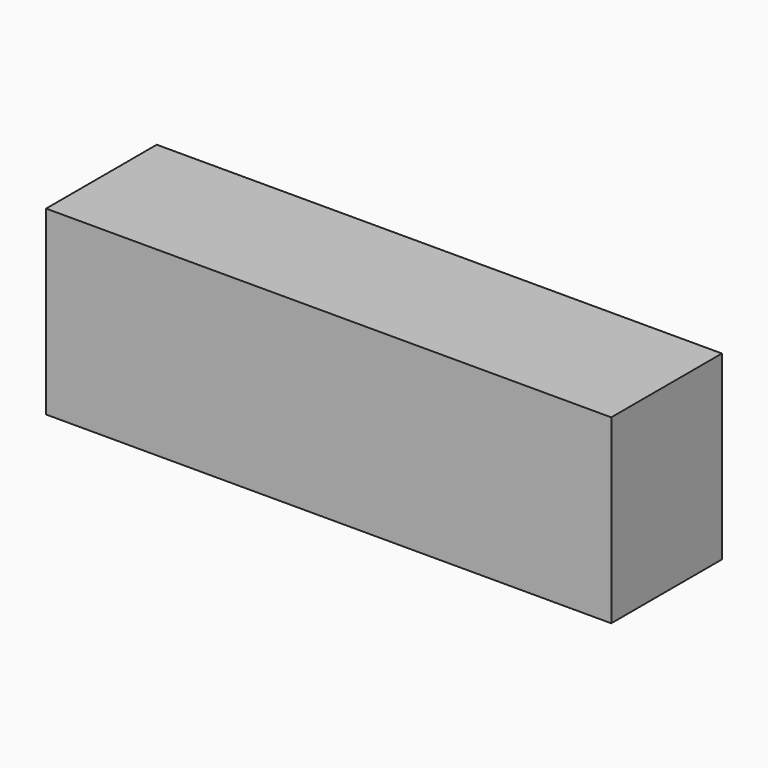
from build123d import *

# Parameters (mm, degrees)
F0_W     = 103.7806421518
F0_H     = 33.2949464209
F1_DEPTH = 25.4


# Not quite as in the source:
# - a feature names something its author has since deleted; it is built from what else it names


with BuildPart() as f1:
    # F0 (on Front) → F1 (new body)
    with BuildSketch(Plane.XZ):
        with Locations((13.251170516, 23.1319440063)):
            Rectangle(F0_W, F0_H)
    extrude(amount=F1_DEPTH)


solid = f1.part
